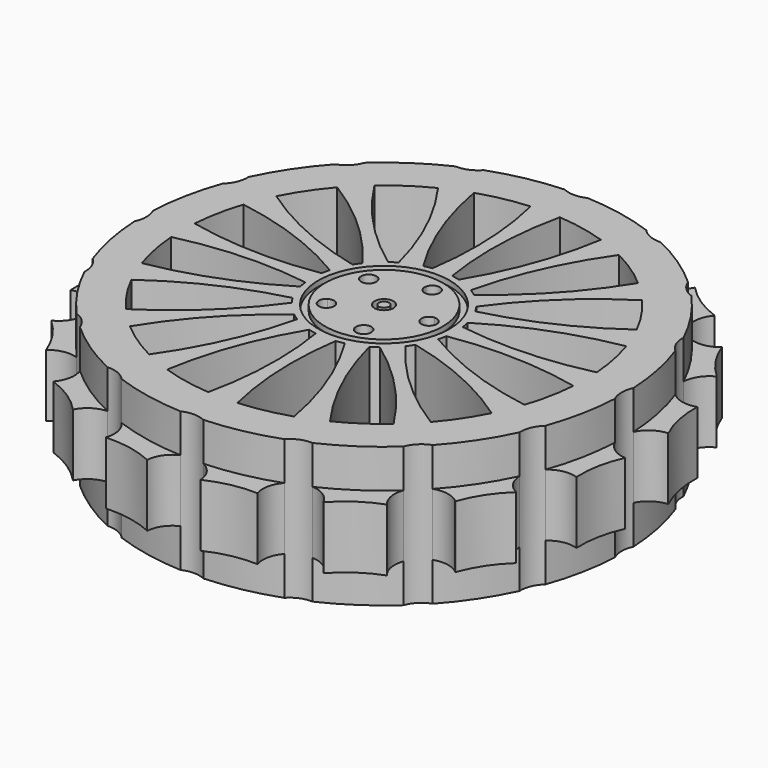
from build123d import *

# Parameters (mm, degrees)
F3_DEPTH  = 30.751
F5_DEPTH  = 20.801
F7_DEPTH  = 1.5
F6_R      = 9.7732794043
F6_R_2    = 8.7701539323
F8_DEPTH  = 0.8
F6_R_3    = 1.4109010528
F6_R_4    = 0.7822608286
F9_DEPTH  = 1.5
F10_DEPTH = 30.751


with BuildPart() as f1:
    # F0 (on Front) → F1 (revolve)
    with BuildSketch(Plane.XZ):
        Polygon((15.6630596573, 13.3769841367), (-20.1369403427, 13.3769841367), (-20.1369403427, 7.6269841367), (-18.1369403427, 7.6269841367), (-18.1369403427, -17.3730158633), (-14.1369403427, -17.3730158633), (-14.1369403427, -7.4230158633), (15.6630596573, -7.4230158633), (15.6630596573, -1.6730158633), (19.1630596573, -1.6730158633), (19.1630596573, 7.6269841367), (15.6630596573, 7.6269841367), align=None)
    revolve(axis=Axis((-20.1369403427, 0, 10.5019841367), (0, 0, -1)))

    # F2 (on face) → F3 (cut, through all)
    with BuildSketch(Plane.XY.offset(13.3769841367)):
        with BuildLine():
            ThreePointArc((18.9510825218, -3.9897850102), (19.0031496784, -3.8784203653), (19.0561068276, -3.7674761754))
            ThreePointArc((19.0561068276, -3.7674761754), (19.1915759594, -1.8859026221), (19.2367669151, 0))
            ThreePointArc((19.2367669151, 0), (19.1859387892, 2), (19.0335856412, 3.9948363383))
            ThreePointArc((19.0335856412, 3.9948363383), (19.0203353599, 3.9941403808), (19.0070874601, 3.9934004743))
            ThreePointArc((19.0070874601, 3.9934004743), (17.0018080089, 3.3173722564), (15.6220600073, 1.7128613401))
            ThreePointArc((15.6220600073, 1.7128613401), (15.652808277, 0.8566759804), (15.6630596573, 0))
            ThreePointArc((15.6630596573, 0), (15.652808277, -0.8566759804), (15.6220600073, -1.7128613401))
            ThreePointArc((15.6220600073, -1.7128613401), (16.9785910085, -3.3016119661), (18.9510825218, -3.9897850102))
        make_face()
        with BuildLine():
            ThreePointArc((19.2367669151, 0), (19.1915759594, -1.8859026221), (19.0561068276, -3.7674761754))
            ThreePointArc((19.0561068276, -3.7674761754), (19.0450111469, -3.8811725923), (19.0335856412, -3.9948363383))
            ThreePointArc((19.0335856412, -3.9948363383), (21.9924224546, -2.8993727853), (23.2367669151, 0))
            ThreePointArc((23.2367669151, 0), (21.9924224546, 2.8993727853), (19.0335856412, 3.9948363383))
            ThreePointArc((19.0335856412, 3.9948363383), (19.1859387892, 2), (19.2367669151, 0))
        make_face()
        with BuildLine():
            ThreePointArc((17.5806645732, -11.2991638023), (18.4802121707, -7.6814292279), (19.0335856412, -3.9948363383))
            ThreePointArc((19.0335856412, -3.9948363383), (18.9923210333, -3.9925237896), (18.9510825218, -3.9897850102))
            ThreePointArc((18.9510825218, -3.9897850102), (17.80492248, -7.5543523288), (17.5556339646, -11.2903499529))
            ThreePointArc((17.5556339646, -11.2903499529), (17.5681565781, -11.2947361201), (17.5806645732, -11.2991638023))
        make_face()
        with BuildLine():
            ThreePointArc((19.0070874601, 3.9934004743), (19.0203353599, 3.9941403808), (19.0335856412, 3.9948363383))
            ThreePointArc((19.0335856412, 3.9948363383), (18.4802121707, 7.6814292279), (17.5806645732, 11.2991638023))
            ThreePointArc((17.5806645732, 11.2991638023), (17.5416560725, 11.285509037), (17.5025085702, 11.2722580441))
            ThreePointArc((17.5025085702, 11.2722580441), (17.8076956231, 7.5404107973), (19.0070874601, 3.9934004743))
        make_face()
        with BuildLine():
            ThreePointArc((20.2396219119, -15.0676654384), (19.5079678731, -12.7616050147), (17.5806645732, -11.2991638023))
            ThreePointArc((17.5806645732, -11.2991638023), (16.283185196, -14.9620613209), (14.6309630405, -18.4792239437))
            ThreePointArc((14.6309630405, -18.4792239437), (14.5772022331, -18.580019603), (14.5231492098, -18.6806588598))
            ThreePointArc((14.5231492098, -18.6806588598), (18.3766887325, -18.4489293151), (20.2396219119, -15.0676654384))
        make_face()
        with BuildLine():
            ThreePointArc((14.6309630405, -18.4792239437), (16.283185196, -14.9620613209), (17.5806645732, -11.2991638023))
            ThreePointArc((17.5806645732, -11.2991638023), (17.5681565781, -11.2947361201), (17.5556339646, -11.2903499529))
            ThreePointArc((17.5556339646, -11.2903499529), (15.444292524, -11.1475313635), (13.5555518405, -12.1018994577))
            ThreePointArc((13.5555518405, -12.1018994577), (12.9379469212, -13.7000668787), (12.2445845269, -15.2668545261))
            ThreePointArc((12.2445845269, -15.2668545261), (12.8898672114, -17.2537906513), (14.448859326, -18.6444194642))
            ThreePointArc((14.448859326, -18.6444194642), (14.5395805109, -18.5614571863), (14.6309630405, -18.4792239437))
        make_face()
        with BuildLine():
            ThreePointArc((15.6220600073, 1.7128613401), (15.2367669151, 0), (15.6220600073, -1.7128613401))
            ThreePointArc((15.6220600073, -1.7128613401), (15.652808277, -0.8566759804), (15.6630596573, 0))
            ThreePointArc((15.6630596573, 0), (15.652808277, 0.8566759804), (15.6220600073, 1.7128613401))
        make_face()
        with BuildLine():
            ThreePointArc((17.5144644688, 11.5178356883), (17.5477231316, 11.4085477626), (17.5806645732, 11.2991638023))
            ThreePointArc((17.5806645732, 11.2991638023), (19.5079678731, 12.7616050147), (20.2396219119, 15.0676654384))
            ThreePointArc((20.2396219119, 15.0676654384), (18.3766887325, 18.4489293151), (14.5231492098, 18.6806588598))
            ThreePointArc((14.5231492098, 18.6806588598), (16.1957524179, 15.1731427195), (17.5144644688, 11.5178356883))
        make_face()
        with BuildLine():
            ThreePointArc((12.2445845269, -15.2668545261), (12.9379469212, -13.7000668787), (13.5555518405, -12.1018994577))
            ThreePointArc((13.5555518405, -12.1018994577), (12.5441037818, -13.5369317089), (12.2445845269, -15.2668545261))
        make_face()
        with BuildLine():
            ThreePointArc((17.5025085702, 11.2722580441), (17.507994946, 11.3950707983), (17.5144644688, 11.5178356883))
            ThreePointArc((17.5144644688, 11.5178356883), (16.1957524179, 15.1731427195), (14.5231492098, 18.6806588598))
            ThreePointArc((14.5231492098, 18.6806588598), (14.5111738775, 18.6749452158), (14.499217564, 18.6691918795))
            ThreePointArc((14.499217564, 18.6691918795), (12.9052857209, 17.2772360224), (12.2445845269, 15.2668545261))
            ThreePointArc((12.2445845269, 15.2668545261), (12.9379469212, 13.7000668787), (13.5555518405, 12.1018994577))
            ThreePointArc((13.5555518405, 12.1018994577), (15.4168116104, 11.1532072117), (17.5025085702, 11.2722580441))
        make_face()
        with BuildLine():
            ThreePointArc((10.3855800677, -24.8729686813), (12.6011007659, -21.8748597161), (14.5231492098, -18.6806588598))
            ThreePointArc((14.5231492098, -18.6806588598), (14.4859106572, -18.6627310616), (14.448859326, -18.6444194642))
            ThreePointArc((14.448859326, -18.6444194642), (12.0258446661, -21.4990337933), (10.365827715, -24.8552469469))
            ThreePointArc((10.365827715, -24.8552469469), (10.3757185877, -24.8640914338), (10.3855800677, -24.8729686813))
        make_face()
        with BuildLine():
            ThreePointArc((12.2445845269, 15.2668545261), (12.5441037818, 13.5369317089), (13.5555518405, 12.1018994577))
            ThreePointArc((13.5555518405, 12.1018994577), (12.9379469212, 13.7000668787), (12.2445845269, 15.2668545261))
        make_face()
        with BuildLine():
            ThreePointArc((14.499217564, 18.6691918795), (14.5111738775, 18.6749452158), (14.5231492098, 18.6806588598))
            ThreePointArc((14.5231492098, 18.6806588598), (12.6011007659, 21.8748597161), (10.3855800677, 24.8729686813))
            ThreePointArc((10.3855800677, 24.8729686813), (10.3547663648, 24.8454254161), (10.3236697241, 24.8182019945))
            ThreePointArc((10.3236697241, 24.8182019945), (12.0337419093, 21.4872147336), (14.499217564, 18.6691918795))
        make_face()
        with BuildLine():
            ThreePointArc((11.7044750597, -27.8414154024), (11.3599107405, -26.2172879493), (10.3855800677, -24.8729686813))
            ThreePointArc((10.3855800677, -24.8729686813), (7.7851352324, -27.7605208669), (4.9127211352, -30.3776773811))
            ThreePointArc((4.9127211352, -30.3776773811), (4.8244797967, -30.4502270574), (4.7360283386, -30.5225204104))
            ThreePointArc((4.7360283386, -30.5225204104), (9.1408268821, -31.5746302961), (11.7044750597, -27.8414154024))
        make_face()
        with BuildLine():
            ThreePointArc((4.9127211352, -30.3776773811), (7.7851352324, -27.7605208669), (10.3855800677, -24.8729686813))
            ThreePointArc((10.3855800677, -24.8729686813), (10.3757185877, -24.8640914338), (10.365827715, -24.8552469469))
            ThreePointArc((10.365827715, -24.8552469469), (8.4698568798, -23.915324386), (6.3596671621, -24.0742557671))
            ThreePointArc((6.3596671621, -24.0742557671), (5.1774824238, -25.3144227665), (3.9373154244, -26.4966075048))
            ThreePointArc((3.9373154244, -26.4966075048), (3.773111353, -28.5792361158), (4.6812616518, -30.4606100668))
            ThreePointArc((4.6812616518, -30.4606100668), (4.7968253868, -30.4186804108), (4.9127211352, -30.3776773811))
        make_face()
        with BuildLine():
            ThreePointArc((3.9373154244, -26.4966075048), (5.1774824238, -25.3144227665), (6.3596671621, -24.0742557671))
            ThreePointArc((6.3596671621, -24.0742557671), (4.876047935, -25.0129882777), (3.9373154244, -26.4966075048))
        make_face()
        with BuildLine():
            ThreePointArc((10.2407370384, 25.0496614779), (10.3132867147, 24.9614201394), (10.3855800677, 24.8729686813))
            ThreePointArc((10.3855800677, 24.8729686813), (11.3599107405, 26.2172879493), (11.7044750597, 27.8414154024))
            ThreePointArc((11.7044750597, 27.8414154024), (9.1408268821, 31.5746302961), (4.7360283386, 30.5225204104))
            ThreePointArc((4.7360283386, 30.5225204104), (7.6235805242, 27.9220755751), (10.2407370384, 25.0496614779))
        make_face()
        with BuildLine():
            ThreePointArc((3.9373154244, 26.4966075048), (5.1774824238, 25.3144227665), (6.3596671621, 24.0742557671))
            ThreePointArc((6.3596671621, 24.0742557671), (8.4422957731, 23.9100516957), (10.3236697241, 24.8182019945))
            ThreePointArc((10.3236697241, 24.8182019945), (10.2817400681, 24.9337657295), (10.2407370384, 25.0496614779))
            ThreePointArc((10.2407370384, 25.0496614779), (7.6235805242, 27.9220755751), (4.7360283386, 30.5225204104))
            ThreePointArc((4.7360283386, 30.5225204104), (4.7271510911, 30.5126589304), (4.7183066042, 30.5027680577))
            ThreePointArc((4.7183066042, 30.5027680577), (3.7783840433, 28.6067972225), (3.9373154244, 26.4966075048))
        make_face()
        with BuildLine():
            ThreePointArc((3.9373154244, 26.4966075048), (4.876047935, 25.0129882777), (6.3596671621, 24.0742557671))
            ThreePointArc((6.3596671621, 24.0742557671), (5.1774824238, 25.3144227665), (3.9373154244, 26.4966075048))
        make_face()
        with BuildLine():
            ThreePointArc((-1.4562814829, -34.6600895525), (1.7379193734, -32.7380411086), (4.7360283386, -30.5225204104))
            ThreePointArc((4.7360283386, -30.5225204104), (4.7084850734, -30.4917067075), (4.6812616518, -30.4606100668))
            ThreePointArc((4.6812616518, -30.4606100668), (1.3502743909, -32.170682252), (-1.4677484632, -34.6361579067))
            ThreePointArc((-1.4677484632, -34.6361579067), (-1.4619951269, -34.6481142202), (-1.4562814829, -34.6600895525))
        make_face()
        with BuildLine():
            ThreePointArc((-8.035040885, -33.6924921832), (-6.436873464, -33.0748872639), (-4.8700858166, -32.3815248696))
            ThreePointArc((-4.8700858166, -32.3815248696), (-6.6000086338, -32.6810441245), (-8.035040885, -33.6924921832))
        make_face()
        with BuildLine():
            ThreePointArc((-1.4677484632, -34.6361579067), (-2.8597043203, -33.0422260636), (-4.8700858166, -32.3815248696))
            ThreePointArc((-4.8700858166, -32.3815248696), (-6.436873464, -33.0748872639), (-8.035040885, -33.6924921832))
            ThreePointArc((-8.035040885, -33.6924921832), (-8.983733131, -35.5537519531), (-8.8646822986, -37.6394489129))
            ThreePointArc((-8.8646822986, -37.6394489129), (-8.7418695444, -37.6449352887), (-8.6191046544, -37.6514048115))
            ThreePointArc((-8.6191046544, -37.6514048115), (-4.9637976232, -36.3326927606), (-1.4562814829, -34.6600895525))
            ThreePointArc((-1.4562814829, -34.6600895525), (-1.4619951269, -34.6481142202), (-1.4677484632, -34.6361579067))
        make_face()
        with BuildLine():
            ThreePointArc((4.7183066042, 30.5027680577), (4.7271510911, 30.5126589304), (4.7360283386, 30.5225204104))
            ThreePointArc((4.7360283386, 30.5225204104), (1.7379193734, 32.7380411086), (-1.4562814829, 34.6600895525))
            ThreePointArc((-1.4562814829, 34.6600895525), (-1.4742092811, 34.6228509999), (-1.4925208785, 34.5857996687))
            ThreePointArc((-1.4925208785, 34.5857996687), (1.3620934506, 32.1627850088), (4.7183066042, 30.5027680577))
        make_face()
        with BuildLine():
            ThreePointArc((-1.0692749043, -36.3765622546), (-1.1672258474, -35.4967820791), (-1.4562814829, -34.6600895525))
            ThreePointArc((-1.4562814829, -34.6600895525), (-4.9637976232, -36.3326927606), (-8.6191046544, -37.6514048115))
            ThreePointArc((-8.6191046544, -37.6514048115), (-8.7283925801, -37.6846634743), (-8.8377765404, -37.7176049159))
            ThreePointArc((-8.8377765404, -37.7176049159), (-4.3888362752, -40.3182628104), (-1.0692749043, -36.3765622546))
        make_face()
        with BuildLine():
            ThreePointArc((-8.035040885, 33.6924921832), (-6.436873464, 33.0748872639), (-4.8700858166, 32.3815248696))
            ThreePointArc((-4.8700858166, 32.3815248696), (-2.8831496914, 33.0268075541), (-1.4925208785, 34.5857996687))
            ThreePointArc((-1.4925208785, 34.5857996687), (-1.5754831564, 34.6765208536), (-1.657716399, 34.7679033832))
            ThreePointArc((-1.657716399, 34.7679033832), (-5.1748790218, 36.4201255387), (-8.8377765404, 37.7176049159))
            ThreePointArc((-8.8377765404, 37.7176049159), (-8.8422042226, 37.7050969208), (-8.8465903898, 37.6925743073))
            ThreePointArc((-8.8465903898, 37.6925743073), (-8.9894089792, 35.5812328667), (-8.035040885, 33.6924921832))
        make_face()
        with BuildLine():
            ThreePointArc((-8.035040885, 33.6924921832), (-6.6000086338, 32.6810441245), (-4.8700858166, 32.3815248696))
            ThreePointArc((-4.8700858166, 32.3815248696), (-6.436873464, 33.0748872639), (-8.035040885, 33.6924921832))
        make_face()
        with BuildLine():
            ThreePointArc((-1.657716399, 34.7679033832), (-1.5569207397, 34.7141425758), (-1.4562814829, 34.6600895525))
            ThreePointArc((-1.4562814829, 34.6600895525), (-1.1672258474, 35.4967820791), (-1.0692749043, 36.3765622546))
            ThreePointArc((-1.0692749043, 36.3765622546), (-4.3888362752, 40.3182628104), (-8.8377765404, 37.7176049159))
            ThreePointArc((-8.8377765404, 37.7176049159), (-5.1748790218, 36.4201255387), (-1.657716399, 34.7679033832))
        make_face()
        with BuildLine():
            ThreePointArc((-8.8377765404, -37.7176049159), (-8.8514313057, -37.6785964152), (-8.8646822986, -37.6394489129))
            ThreePointArc((-8.8646822986, -37.6394489129), (-12.5965295454, -37.9446359658), (-16.1435398684, -39.1440278028))
            ThreePointArc((-16.1435398684, -39.1440278028), (-16.1427999619, -39.1572757026), (-16.1421040044, -39.1705259839))
            ThreePointArc((-16.1421040044, -39.1705259839), (-12.4555111148, -38.6171525134), (-8.8377765404, -37.7176049159))
        make_face()
        with BuildLine():
            ThreePointArc((-21.8498016828, -35.75900035), (-20.1369403427, -35.8), (-18.4240790026, -35.75900035))
            ThreePointArc((-18.4240790026, -35.75900035), (-20.1369403427, -35.3737072578), (-21.8498016828, -35.75900035))
        make_face()
        with BuildLine():
            ThreePointArc((-16.1435398684, -39.1440278028), (-16.8195680863, -37.1387483516), (-18.4240790026, -35.75900035))
            ThreePointArc((-18.4240790026, -35.75900035), (-20.1369403427, -35.8), (-21.8498016828, -35.75900035))
            ThreePointArc((-21.8498016828, -35.75900035), (-23.4385523088, -37.1155313512), (-24.1267253529, -39.0880228645))
            ThreePointArc((-24.1267253529, -39.0880228645), (-24.015360708, -39.1400900211), (-23.9044165181, -39.1930471703))
            ThreePointArc((-23.9044165181, -39.1930471703), (-20.022703913, -39.3735415382), (-16.1421040044, -39.1705259839))
            ThreePointArc((-16.1421040044, -39.1705259839), (-16.1427999619, -39.1572757026), (-16.1435398684, -39.1440278028))
        make_face()
        with BuildLine():
            ThreePointArc((-16.1471553325, 39.0880228645), (-12.5825880139, 37.9418628227), (-8.8465903898, 37.6925743073))
            ThreePointArc((-8.8465903898, 37.6925743073), (-8.8422042226, 37.7050969208), (-8.8377765404, 37.7176049159))
            ThreePointArc((-8.8377765404, 37.7176049159), (-12.4555111148, 38.6171525134), (-16.1421040044, 39.1705259839))
            ThreePointArc((-16.1421040044, 39.1705259839), (-16.1444165531, 39.129261376), (-16.1471553325, 39.0880228645))
        make_face()
        with BuildLine():
            ThreePointArc((-21.8498016828, 35.75900035), (-20.1369403427, 35.8), (-18.4240790026, 35.75900035))
            ThreePointArc((-18.4240790026, 35.75900035), (-16.8353283766, 37.1155313512), (-16.1471553325, 39.0880228645))
            ThreePointArc((-16.1471553325, 39.0880228645), (-16.2585199774, 39.1400900211), (-16.3694641673, 39.1930471703))
            ThreePointArc((-16.3694641673, 39.1930471703), (-20.2511767724, 39.3735415382), (-24.131776681, 39.1705259839))
            ThreePointArc((-24.131776681, 39.1705259839), (-24.1310807235, 39.1572757026), (-24.130340817, 39.1440278028))
            ThreePointArc((-24.130340817, 39.1440278028), (-23.4543125991, 37.1387483516), (-21.8498016828, 35.75900035))
        make_face()
        with BuildLine():
            ThreePointArc((-21.8498016828, 35.75900035), (-20.1369403427, 35.3737072578), (-18.4240790026, 35.75900035))
            ThreePointArc((-18.4240790026, 35.75900035), (-20.1369403427, 35.8), (-21.8498016828, 35.75900035))
        make_face()
        with BuildLine():
            ThreePointArc((-16.1369403427, -39.3737072578), (-16.1382314665, -39.2720838187), (-16.1421040044, -39.1705259839))
            ThreePointArc((-16.1421040044, -39.1705259839), (-20.022703913, -39.3735415382), (-23.9044165181, -39.1930471703))
            ThreePointArc((-23.9044165181, -39.1930471703), (-24.018112935, -39.1819514896), (-24.131776681, -39.1705259839))
            ThreePointArc((-24.131776681, -39.1705259839), (-20.2385637818, -43.372416134), (-16.1369403427, -39.3737072578))
        make_face()
        with BuildLine():
            ThreePointArc((-24.131776681, -39.1705259839), (-24.1294641323, -39.129261376), (-24.1267253529, -39.0880228645))
            ThreePointArc((-24.1267253529, -39.0880228645), (-27.6912926715, -37.9418628227), (-31.4272902956, -37.6925743073))
            ThreePointArc((-31.4272902956, -37.6925743073), (-31.4316764628, -37.7050969208), (-31.436104145, -37.7176049159))
            ThreePointArc((-31.436104145, -37.7176049159), (-27.8183695706, -38.6171525134), (-24.131776681, -39.1705259839))
        make_face()
        with BuildLine():
            ThreePointArc((-35.4037948688, -32.3815248696), (-33.8370072214, -33.0748872639), (-32.2388398004, -33.6924921832))
            ThreePointArc((-32.2388398004, -33.6924921832), (-33.6738720516, -32.6810441245), (-35.4037948688, -32.3815248696))
        make_face()
        with BuildLine():
            ThreePointArc((-31.2046057811, -36.3765622546), (-31.4721090347, -34.9383452895), (-32.2388398004, -33.6924921832))
            ThreePointArc((-32.2388398004, -33.6924921832), (-33.8370072214, -33.0748872639), (-35.4037948688, -32.3815248696))
            ThreePointArc((-35.4037948688, -32.3815248696), (-37.390730994, -33.0268075541), (-38.7813598069, -34.5857996687))
            ThreePointArc((-38.7813598069, -34.5857996687), (-38.698397529, -34.6765208536), (-38.6161642864, -34.7679033832))
            ThreePointArc((-38.6161642864, -34.7679033832), (-35.0990016636, -36.4201255387), (-31.436104145, -37.7176049159))
            ThreePointArc((-31.436104145, -37.7176049159), (-31.4316764628, -37.7050969208), (-31.4272902956, -37.6925743073))
            ThreePointArc((-31.4272902956, -37.6925743073), (-31.2606698065, -37.0439219994), (-31.2046057811, -36.3765622546))
        make_face()
        with BuildLine():
            ThreePointArc((-16.3694641673, 39.1930471703), (-16.2557677504, 39.1819514896), (-16.1421040044, 39.1705259839))
            ThreePointArc((-16.1421040044, 39.1705259839), (-16.1382314665, 39.2720838187), (-16.1369403427, 39.3737072578))
            ThreePointArc((-16.1369403427, 39.3737072578), (-20.2385637818, 43.372416134), (-24.131776681, 39.1705259839))
            ThreePointArc((-24.131776681, 39.1705259839), (-20.2511767724, 39.3735415382), (-16.3694641673, 39.1930471703))
        make_face()
        with BuildLine():
            ThreePointArc((-31.4091983868, 37.6394489129), (-27.67735114, 37.9446359658), (-24.130340817, 39.1440278028))
            ThreePointArc((-24.130340817, 39.1440278028), (-24.1310807235, 39.1572757026), (-24.131776681, 39.1705259839))
            ThreePointArc((-24.131776681, 39.1705259839), (-27.8183695706, 38.6171525134), (-31.436104145, 37.7176049159))
            ThreePointArc((-31.436104145, 37.7176049159), (-31.4224493797, 37.6785964152), (-31.4091983868, 37.6394489129))
        make_face()
        with BuildLine():
            ThreePointArc((-35.4037948688, 32.3815248696), (-33.8370072214, 33.0748872639), (-32.2388398004, 33.6924921832))
            ThreePointArc((-32.2388398004, 33.6924921832), (-31.4721090347, 34.9383452895), (-31.2046057811, 36.3765622546))
            ThreePointArc((-31.2046057811, 36.3765622546), (-31.2560851988, 37.016238119), (-31.4091983868, 37.6394489129))
            ThreePointArc((-31.4091983868, 37.6394489129), (-31.532011141, 37.6449352887), (-31.654776031, 37.6514048115))
            ThreePointArc((-31.654776031, 37.6514048115), (-35.3100830622, 36.3326927606), (-38.8175992025, 34.6600895525))
            ThreePointArc((-38.8175992025, 34.6600895525), (-38.8118855585, 34.6481142202), (-38.8061322222, 34.6361579067))
            ThreePointArc((-38.8061322222, 34.6361579067), (-37.4141763651, 33.0422260636), (-35.4037948688, 32.3815248696))
        make_face()
        with BuildLine():
            ThreePointArc((-35.4037948688, 32.3815248696), (-33.6738720516, 32.6810441245), (-32.2388398004, 33.6924921832))
            ThreePointArc((-32.2388398004, 33.6924921832), (-33.8370072214, 33.0748872639), (-35.4037948688, 32.3815248696))
        make_face()
        with BuildLine():
            ThreePointArc((-38.8175992025, -34.6600895525), (-36.7353395105, -40.0720803846), (-31.436104145, -37.7176049159))
            ThreePointArc((-31.436104145, -37.7176049159), (-35.0990016636, -36.4201255387), (-38.6161642864, -34.7679033832))
            ThreePointArc((-38.6161642864, -34.7679033832), (-38.7169599457, -34.7141425758), (-38.8175992025, -34.6600895525))
        make_face()
        with BuildLine():
            ThreePointArc((-38.8175992025, -34.6600895525), (-38.7996714043, -34.6228509999), (-38.7813598069, -34.5857996687))
            ThreePointArc((-38.7813598069, -34.5857996687), (-41.635974136, -32.1627850088), (-44.9921872896, -30.5027680577))
            ThreePointArc((-44.9921872896, -30.5027680577), (-45.0010317765, -30.5126589304), (-45.009909024, -30.5225204104))
            ThreePointArc((-45.009909024, -30.5225204104), (-42.0118000588, -32.7380411086), (-38.8175992025, -34.6600895525))
        make_face()
        with BuildLine():
            ThreePointArc((-46.6335478475, -24.0742557671), (-45.4513631092, -25.3144227665), (-44.2111961098, -26.4966075048))
            ThreePointArc((-44.2111961098, -26.4966075048), (-45.1499286204, -25.0129882777), (-46.6335478475, -24.0742557671))
        make_face()
        with BuildLine():
            ThreePointArc((-43.9783557451, -27.8414154024), (-44.0369956663, -27.1590073652), (-44.2111961098, -26.4966075048))
            ThreePointArc((-44.2111961098, -26.4966075048), (-45.4513631092, -25.3144227665), (-46.6335478475, -24.0742557671))
            ThreePointArc((-46.6335478475, -24.0742557671), (-48.7161764585, -23.9100516957), (-50.5975504095, -24.8182019945))
            ThreePointArc((-50.5975504095, -24.8182019945), (-50.5556207535, -24.9337657295), (-50.5146177238, -25.0496614779))
            ThreePointArc((-50.5146177238, -25.0496614779), (-47.8974612096, -27.9220755751), (-45.009909024, -30.5225204104))
            ThreePointArc((-45.009909024, -30.5225204104), (-45.0010317765, -30.5126589304), (-44.9921872896, -30.5027680577))
            ThreePointArc((-44.9921872896, -30.5027680577), (-44.240396822, -29.2653757562), (-43.9783557451, -27.8414154024))
        make_face()
        with BuildLine():
            ThreePointArc((-31.654776031, 37.6514048115), (-31.5454881053, 37.6846634743), (-31.436104145, 37.7176049159))
            ThreePointArc((-31.436104145, 37.7176049159), (-36.7353395105, 40.0720803846), (-38.8175992025, 34.6600895525))
            ThreePointArc((-38.8175992025, 34.6600895525), (-35.3100830622, 36.3326927606), (-31.654776031, 37.6514048115))
        make_face()
        with BuildLine():
            ThreePointArc((-44.9551423372, 30.4606100668), (-41.6241550763, 32.170682252), (-38.8061322222, 34.6361579067))
            ThreePointArc((-38.8061322222, 34.6361579067), (-38.8118855585, 34.6481142202), (-38.8175992025, 34.6600895525))
            ThreePointArc((-38.8175992025, 34.6600895525), (-42.0118000588, 32.7380411086), (-45.009909024, 30.5225204104))
            ThreePointArc((-45.009909024, 30.5225204104), (-44.9823657588, 30.4917067075), (-44.9551423372, 30.4606100668))
        make_face()
        with BuildLine():
            ThreePointArc((-46.6335478475, 24.0742557671), (-45.4513631092, 25.3144227665), (-44.2111961098, 26.4966075048))
            ThreePointArc((-44.2111961098, 26.4966075048), (-44.0369956663, 27.1590073652), (-43.9783557451, 27.8414154024))
            ThreePointArc((-43.9783557451, 27.8414154024), (-44.2304994491, 29.2391182264), (-44.9551423372, 30.4606100668))
            ThreePointArc((-44.9551423372, 30.4606100668), (-45.0707060722, 30.4186804108), (-45.1866018206, 30.3776773811))
            ThreePointArc((-45.1866018206, 30.3776773811), (-48.0590159178, 27.7605208669), (-50.6594607531, 24.8729686813))
            ThreePointArc((-50.6594607531, 24.8729686813), (-50.6495992731, 24.8640914338), (-50.6397084004, 24.8552469469))
            ThreePointArc((-50.6397084004, 24.8552469469), (-48.7437375652, 23.915324386), (-46.6335478475, 24.0742557671))
        make_face()
        with BuildLine():
            ThreePointArc((-46.6335478475, 24.0742557671), (-45.1499286204, 25.0129882777), (-44.2111961098, 26.4966075048))
            ThreePointArc((-44.2111961098, 26.4966075048), (-45.4513631092, 25.3144227665), (-46.6335478475, 24.0742557671))
        make_face()
        with BuildLine():
            ThreePointArc((-50.6594607531, -24.8729686813), (-50.8067828699, -30.6698425272), (-45.009909024, -30.5225204104))
            ThreePointArc((-45.009909024, -30.5225204104), (-47.8974612096, -27.9220755751), (-50.5146177238, -25.0496614779))
            ThreePointArc((-50.5146177238, -25.0496614779), (-50.5871674001, -24.9614201394), (-50.6594607531, -24.8729686813))
        make_face()
        with BuildLine():
            ThreePointArc((-50.6594607531, -24.8729686813), (-50.6286470502, -24.8454254161), (-50.5975504095, -24.8182019945))
            ThreePointArc((-50.5975504095, -24.8182019945), (-52.3076225947, -21.4872147336), (-54.7730982494, -18.6691918795))
            ThreePointArc((-54.7730982494, -18.6691918795), (-54.7850545629, -18.6749452158), (-54.7970298952, -18.6806588598))
            ThreePointArc((-54.7970298952, -18.6806588598), (-52.8749814513, -21.8748597161), (-50.6594607531, -24.8729686813))
        make_face()
        with BuildLine():
            ThreePointArc((-53.8294325259, -12.1018994577), (-53.2118276066, -13.7000668787), (-52.5184652123, -15.2668545261))
            ThreePointArc((-52.5184652123, -15.2668545261), (-52.5147434435, -15.1672908872), (-52.5135025973, -15.0676654384))
            ThreePointArc((-52.5135025973, -15.0676654384), (-52.8572558684, -13.4453646471), (-53.8294325259, -12.1018994577))
        make_face()
        with BuildLine():
            ThreePointArc((-54.7730982494, -18.6691918795), (-53.1791664063, -17.2772360224), (-52.5184652123, -15.2668545261))
            ThreePointArc((-52.5184652123, -15.2668545261), (-53.2118276066, -13.7000668787), (-53.8294325259, -12.1018994577))
            ThreePointArc((-53.8294325259, -12.1018994577), (-55.6906922958, -11.1532072117), (-57.7763892556, -11.2722580441))
            ThreePointArc((-57.7763892556, -11.2722580441), (-57.7818756314, -11.3950707983), (-57.7883451542, -11.5178356883))
            ThreePointArc((-57.7883451542, -11.5178356883), (-56.4696331033, -15.1731427195), (-54.7970298952, -18.6806588598))
            ThreePointArc((-54.7970298952, -18.6806588598), (-54.7850545629, -18.6749452158), (-54.7730982494, -18.6691918795))
        make_face()
        with BuildLine():
            ThreePointArc((-45.1866018206, 30.3776773811), (-45.0983604821, 30.4502270574), (-45.009909024, 30.5225204104))
            ThreePointArc((-45.009909024, 30.5225204104), (-50.8067828699, 30.6698425272), (-50.6594607531, 24.8729686813))
            ThreePointArc((-50.6594607531, 24.8729686813), (-48.0590159178, 27.7605208669), (-45.1866018206, 30.3776773811))
        make_face()
        with BuildLine():
            ThreePointArc((-54.7227400114, 18.6444194642), (-52.2997253515, 21.4990337933), (-50.6397084004, 24.8552469469))
            ThreePointArc((-50.6397084004, 24.8552469469), (-50.6495992731, 24.8640914338), (-50.6594607531, 24.8729686813))
            ThreePointArc((-50.6594607531, 24.8729686813), (-52.8749814513, 21.8748597161), (-54.7970298952, 18.6806588598))
            ThreePointArc((-54.7970298952, 18.6806588598), (-54.7597913426, 18.6627310616), (-54.7227400114, 18.6444194642))
        make_face()
        with BuildLine():
            ThreePointArc((-53.8294325259, 12.1018994577), (-53.2118276066, 13.7000668787), (-52.5184652123, 15.2668545261))
            ThreePointArc((-52.5184652123, 15.2668545261), (-53.1637478968, 17.2537906513), (-54.7227400114, 18.6444194642))
            ThreePointArc((-54.7227400114, 18.6444194642), (-54.8134611963, 18.5614571863), (-54.9048437259, 18.4792239437))
            ThreePointArc((-54.9048437259, 18.4792239437), (-56.5570658814, 14.9620613209), (-57.8545452586, 11.2991638023))
            ThreePointArc((-57.8545452586, 11.2991638023), (-57.8420372635, 11.2947361201), (-57.82951465, 11.2903499529))
            ThreePointArc((-57.82951465, 11.2903499529), (-55.7181732094, 11.1475313635), (-53.8294325259, 12.1018994577))
        make_face()
        with BuildLine():
            ThreePointArc((-52.5135025973, 15.0676654384), (-52.5147434435, 15.1672908872), (-52.5184652123, 15.2668545261))
            ThreePointArc((-52.5184652123, 15.2668545261), (-53.2118276066, 13.7000668787), (-53.8294325259, 12.1018994577))
            ThreePointArc((-53.8294325259, 12.1018994577), (-52.8572558684, 13.4453646471), (-52.5135025973, 15.0676654384))
        make_face()
        with BuildLine():
            ThreePointArc((-57.8545452586, -11.2991638023), (-60.2090207273, -16.5983991678), (-54.7970298952, -18.6806588598))
            ThreePointArc((-54.7970298952, -18.6806588598), (-56.4696331033, -15.1731427195), (-57.7883451542, -11.5178356883))
            ThreePointArc((-57.7883451542, -11.5178356883), (-57.821603817, -11.4085477626), (-57.8545452586, -11.2991638023))
        make_face()
        with BuildLine():
            ThreePointArc((-57.8545452586, -11.2991638023), (-57.8155367579, -11.285509037), (-57.7763892556, -11.2722580441))
            ThreePointArc((-57.7763892556, -11.2722580441), (-58.0815763085, -7.5404107973), (-59.2809681455, -3.9934004743))
            ThreePointArc((-59.2809681455, -3.9934004743), (-59.2942160453, -3.9941403808), (-59.3074663266, -3.9948363383))
            ThreePointArc((-59.3074663266, -3.9948363383), (-58.7540928561, -7.6814292279), (-57.8545452586, -11.2991638023))
        make_face()
        with BuildLine():
            ThreePointArc((-55.8959406927, 1.7128613401), (-55.9369403427, 0), (-55.8959406927, -1.7128613401))
            ThreePointArc((-55.8959406927, -1.7128613401), (-55.6081594435, -0.8778303847), (-55.5106476005, 0))
            ThreePointArc((-55.5106476005, 0), (-55.6081594435, 0.8778303847), (-55.8959406927, 1.7128613401))
        make_face()
        with BuildLine():
            ThreePointArc((-59.2809681455, -3.9934004743), (-57.2756886943, -3.3173722564), (-55.8959406927, -1.7128613401))
            ThreePointArc((-55.8959406927, -1.7128613401), (-55.9369403427, 0), (-55.8959406927, 1.7128613401))
            ThreePointArc((-55.8959406927, 1.7128613401), (-57.2524716939, 3.3016119661), (-59.2249632072, 3.9897850102))
            ThreePointArc((-59.2249632072, 3.9897850102), (-59.2770303638, 3.8784203653), (-59.329987513, 3.7674761754))
            ThreePointArc((-59.329987513, 3.7674761754), (-59.5104818809, -0.1142364297), (-59.3074663266, -3.9948363383))
            ThreePointArc((-59.3074663266, -3.9948363383), (-59.2942160453, -3.9941403808), (-59.2809681455, -3.9934004743))
        make_face()
        with BuildLine():
            ThreePointArc((-54.9048437259, 18.4792239437), (-54.8510829185, 18.580019603), (-54.7970298952, 18.6806588598))
            ThreePointArc((-54.7970298952, 18.6806588598), (-60.2090207273, 16.5983991678), (-57.8545452586, 11.2991638023))
            ThreePointArc((-57.8545452586, 11.2991638023), (-56.5570658814, 14.9620613209), (-54.9048437259, 18.4792239437))
        make_face()
        with BuildLine():
            ThreePointArc((-59.2249632072, 3.9897850102), (-58.0788031654, 7.5543523288), (-57.82951465, 11.2903499529))
            ThreePointArc((-57.82951465, 11.2903499529), (-57.8420372635, 11.2947361201), (-57.8545452586, 11.2991638023))
            ThreePointArc((-57.8545452586, 11.2991638023), (-58.7540928561, 7.6814292279), (-59.3074663266, 3.9948363383))
            ThreePointArc((-59.3074663266, 3.9948363383), (-59.2662017187, 3.9925237896), (-59.2249632072, 3.9897850102))
        make_face()
        with BuildLine():
            ThreePointArc((-59.3074663266, 3.9948363383), (-63.5106476005, 0), (-59.3074663266, -3.9948363383))
            ThreePointArc((-59.3074663266, -3.9948363383), (-59.5104818809, -0.1142364297), (-59.329987513, 3.7674761754))
            ThreePointArc((-59.329987513, 3.7674761754), (-59.3188918323, 3.8811725923), (-59.3074663266, 3.9948363383))
        make_face()
    extrude(amount=-F3_DEPTH, mode=Mode.SUBTRACT)

    # F4 (on face) → F5 (cut, through all)
    with BuildSketch(Plane(origin=(0, 0, -7.4230158633), x_dir=(1, 0, 0), z_dir=(0, 0, -1))):
        with BuildLine():
            ThreePointArc((-11.6660608479, 6.6032522858), (-11.3052466368, 6.1122766994), (-10.9728543085, 5.6016307735))
            ThreePointArc((-10.9728543085, 5.6016307735), (-1.7575267031, 8.7043382506), (6.6978225975, 13.5060176204))
            ThreePointArc((6.6978225975, 13.5060176204), (4.8243988213, 16.7167150229), (2.5687959513, 19.6714654605))
            ThreePointArc((2.5687959513, 19.6714654605), (-5.1757327792, 13.8204425733), (-11.6660608479, 6.6032522858))
        make_face()
        with BuildLine():
            ThreePointArc((-9.7839129056, 2.8589443946), (-9.6384522635, 2.2672644786), (-9.5267775303, 1.6682881223))
            ThreePointArc((-9.5267775303, 1.6682881223), (0.1744297767, 1.0082628574), (9.8236770781, 2.2087140565))
            ThreePointArc((9.8236770781, 2.2087140565), (9.3215398978, 5.8919399127), (8.368368612, 9.484955214))
            ThreePointArc((8.368368612, 9.484955214), (-1.0257324924, 7.043017761), (-9.7839129056, 2.8589443946))
        make_face()
        with BuildLine():
            ThreePointArc((9.8282663856, -2.1455534824), (0.2147596427, -0.8066426603), (-9.4779195402, -1.3206118642))
            ThreePointArc((-9.4779195402, -1.3206118642), (-9.5699575313, -1.9229182062), (-9.6960018589, -2.5190362725))
            ThreePointArc((-9.6960018589, -2.5190362725), (-0.9858357211, -6.841311416), (8.38829915, -9.4248462004))
            ThreePointArc((8.38829915, -9.4248462004), (9.3338943995, -5.8298296385), (9.8282663856, -2.1455534824))
        make_face()
        with BuildLine():
            ThreePointArc((6.7262330701, -13.4494211106), (-1.6431100563, -8.5334990488), (-10.7946654676, -5.2991169381))
            ThreePointArc((-10.7946654676, -5.2991169381), (-11.1101901421, -5.8203540254), (-11.4547644243, -6.3228602299))
            ThreePointArc((-11.4547644243, -6.3228602299), (-5.0616832924, -13.649358043), (2.6102120911, -19.6235590597))
            ThreePointArc((2.6102120911, -19.6235590597), (4.8595814655, -16.6640604749), (6.7262330701, -13.4494211106))
        make_face()
        with BuildLine():
            ThreePointArc((-0.4654748822, -22.705736294), (-6.3164977694, -14.9612075635), (-13.5336880569, -8.4708794948))
            ThreePointArc((-13.5336880569, -8.4708794948), (-14.0246636433, -8.8316937059), (-14.5353095692, -9.1640860342))
            ThreePointArc((-14.5353095692, -9.1640860342), (-11.4326020921, -18.3794136396), (-6.6309227223, -26.8347629402))
            ThreePointArc((-6.6309227223, -26.8347629402), (-3.4202253198, -24.961339164), (-0.4654748822, -22.705736294))
        make_face()
        with BuildLine():
            ThreePointArc((-10.6519851287, -28.5053089547), (-13.0939225817, -19.1112078503), (-17.2779959481, -10.3530274371))
            ThreePointArc((-17.2779959481, -10.3530274371), (-17.8696758641, -10.4984880792), (-18.4686522204, -10.6101628124))
            ThreePointArc((-18.4686522204, -10.6101628124), (-19.1286774853, -20.3113701194), (-17.9282262862, -29.9606174208))
            ThreePointArc((-17.9282262862, -29.9606174208), (-14.24500043, -29.4584802405), (-10.6519851287, -28.5053089547))
        make_face()
        with BuildLine():
            ThreePointArc((-22.2824938251, -29.9652067283), (-20.943583003, -20.3516999854), (-21.4575522069, -10.6590208025))
            ThreePointArc((-21.4575522069, -10.6590208025), (-22.0598585489, -10.5669828114), (-22.6559766152, -10.4409384838))
            ThreePointArc((-22.6559766152, -10.4409384838), (-26.9782517587, -19.1511046216), (-29.5617865431, -28.5252394927))
            ThreePointArc((-29.5617865431, -28.5252394927), (-25.9667699812, -29.4708347422), (-22.2824938251, -29.9652067283))
        make_face()
        with BuildLine():
            ThreePointArc((-42.8426766367, -19.6714654605), (-35.0981479062, -13.8204425733), (-28.6078198375, -6.6032522858))
            ThreePointArc((-28.6078198375, -6.6032522858), (-28.9686340486, -6.1122766994), (-29.3010263769, -5.6016307735))
            ThreePointArc((-29.3010263769, -5.6016307735), (-38.5163539823, -8.7043382506), (-46.9717032829, -13.5060176204))
            ThreePointArc((-46.9717032829, -13.5060176204), (-45.0982795067, -16.7167150229), (-42.8426766367, -19.6714654605))
        make_face()
        with BuildLine():
            ThreePointArc((-48.6422492974, -9.484955214), (-39.248148193, -7.043017761), (-30.4899677798, -2.8589443946))
            ThreePointArc((-30.4899677798, -2.8589443946), (-30.6354284219, -2.2672644786), (-30.7471031551, -1.6682881223))
            ThreePointArc((-30.7471031551, -1.6682881223), (-40.4483104621, -1.0082628574), (-50.0975577635, -2.2087140565))
            ThreePointArc((-50.0975577635, -2.2087140565), (-49.5954205832, -5.8919399127), (-48.6422492974, -9.484955214))
        make_face()
        with BuildLine():
            ThreePointArc((-30.7959611452, 1.3206118642), (-30.7039231541, 1.9229182062), (-30.5778788265, 2.5190362725))
            ThreePointArc((-30.5778788265, 2.5190362725), (-39.2880449643, 6.841311416), (-48.6621798354, 9.4248462004))
            ThreePointArc((-48.6621798354, 9.4248462004), (-49.6077750849, 5.8298296385), (-50.102147071, 2.1455534824))
            ThreePointArc((-50.102147071, 2.1455534824), (-40.4886403281, 0.8066426603), (-30.7959611452, 1.3206118642))
        make_face()
        with BuildLine():
            ThreePointArc((-33.5863614533, -26.8631734128), (-28.6704393915, -18.4938302864), (-25.4360572808, -9.3422748751))
            ThreePointArc((-25.4360572808, -9.3422748751), (-25.9572943681, -9.0267502006), (-26.4598005726, -8.6821759184))
            ThreePointArc((-26.4598005726, -8.6821759184), (-33.7862983857, -15.0752570503), (-39.7604994024, -22.7471524338))
            ThreePointArc((-39.7604994024, -22.7471524338), (-36.8010008176, -24.9965218082), (-33.5863614533, -26.8631734128))
        make_face()
        with BuildLine():
            ThreePointArc((-29.4792152178, 5.2991169381), (-29.1636905433, 5.8203540254), (-28.8191162611, 6.3228602299))
            ThreePointArc((-28.8191162611, 6.3228602299), (-35.212197393, 13.649358043), (-42.8840927765, 19.6235590597))
            ThreePointArc((-42.8840927765, 19.6235590597), (-45.1334621509, 16.6640604749), (-47.0001137555, 13.4494211106))
            ThreePointArc((-47.0001137555, 13.4494211106), (-38.6307706291, 8.5334990488), (-29.4792152178, 5.2991169381))
        make_face()
        with BuildLine():
            ThreePointArc((-26.7401926285, 8.4708794948), (-26.2492170421, 8.8316937059), (-25.7385711162, 9.1640860342))
            ThreePointArc((-25.7385711162, 9.1640860342), (-28.8412785933, 18.3794136396), (-33.6429579631, 26.8347629402))
            ThreePointArc((-33.6429579631, 26.8347629402), (-36.8536553656, 24.961339164), (-39.8084058032, 22.705736294))
            ThreePointArc((-39.8084058032, 22.705736294), (-33.957382916, 14.9612075635), (-26.7401926285, 8.4708794948))
        make_face()
        with BuildLine():
            ThreePointArc((-22.9958847373, 10.3530274371), (-22.4042048213, 10.4984880792), (-21.805228465, 10.6101628124))
            ThreePointArc((-21.805228465, 10.6101628124), (-21.1452032001, 20.3113701194), (-22.3456543992, 29.9606174208))
            ThreePointArc((-22.3456543992, 29.9606174208), (-26.0288802554, 29.4584802405), (-29.6218955567, 28.5053089547))
            ThreePointArc((-29.6218955567, 28.5053089547), (-27.1799581037, 19.1112078503), (-22.9958847373, 10.3530274371))
        make_face()
        with BuildLine():
            ThreePointArc((-18.8163284785, 10.6590208025), (-18.2140221365, 10.5669828114), (-17.6179040702, 10.4409384838))
            ThreePointArc((-17.6179040702, 10.4409384838), (-13.2956289267, 19.1511046216), (-10.7120941424, 28.5252394927))
            ThreePointArc((-10.7120941424, 28.5252394927), (-14.3071107042, 29.4708347422), (-17.9913868603, 29.9652067283))
            ThreePointArc((-17.9913868603, 29.9652067283), (-19.3302976824, 20.3516999854), (-18.8163284785, 10.6590208025))
        make_face()
        with BuildLine():
            ThreePointArc((-14.8378234046, 9.3422748751), (-14.3165863173, 9.0267502006), (-13.8140801128, 8.6821759184))
            ThreePointArc((-13.8140801128, 8.6821759184), (-6.4875822997, 15.0752570503), (-0.513381283, 22.7471524338))
            ThreePointArc((-0.513381283, 22.7471524338), (-3.4728798678, 24.9965218082), (-6.6875192321, 26.8631734128))
            ThreePointArc((-6.6875192321, 26.8631734128), (-11.6034412939, 18.4938302864), (-14.8378234046, 9.3422748751))
        make_face()
    extrude(amount=-F5_DEPTH, mode=Mode.SUBTRACT)

    # F6 (on face) → F7 (cut)
    with BuildSketch(Plane.XY.offset(13.3769841367)):
        with BuildLine():
            ThreePointArc((-26.1477993657, 2.9672449234), (-25.5600684796, 3.9401332263), (-24.8164155515, 4.7997375346))
            ThreePointArc((-24.8164155515, 4.7997375346), (-26.4796255541, 4.6082305478), (-26.1477993657, 2.9672449234))
        make_face()
        with BuildLine():
            ThreePointArc((-19.1723803117, 6.6335957502), (-18.0654897197, 6.3752694803), (-17.0181560482, 5.9336458569))
            ThreePointArc((-17.0181560482, 5.9336458569), (-16.95140368, 6.1499884549), (-16.9288546665, 6.3752694803))
            ThreePointArc((-16.9288546665, 6.3752694803), (-17.9354731875, 7.5044439335), (-19.1723803117, 6.6335957502))
        make_face()
        with BuildLine():
            ThreePointArc((-19.1723803117, 6.6335957502), (-18.4167292676, 5.2942653063), (-17.0181560482, 5.9336458569))
            ThreePointArc((-17.0181560482, 5.9336458569), (-18.0654897197, 6.3752694803), (-19.1723803117, 6.6335957502))
        make_face()
        with BuildLine():
            ThreePointArc((-13.5299504364, -1.1325427178), (-13.4577200425, -0.5683175266), (-13.4335853148, 0))
            ThreePointArc((-13.4335853148, 0), (-13.4577200425, 0.5683175266), (-13.5299504364, 1.1325427178))
            ThreePointArc((-13.5299504364, 1.1325427178), (-14.5702203681, 0), (-13.5299504364, -1.1325427178))
        make_face()
        with BuildLine():
            ThreePointArc((-13.5299504364, 1.1325427178), (-13.4577200425, 0.5683175266), (-13.4335853148, 0))
            ThreePointArc((-13.4335853148, 0), (-13.4577200425, -0.5683175266), (-13.5299504364, -1.1325427178))
            ThreePointArc((-13.5299504364, -1.1325427178), (-12.6646876398, -0.837099522), (-12.2969502615, 0))
            ThreePointArc((-12.2969502615, 0), (-12.6646876398, 0.837099522), (-13.5299504364, 1.1325427178))
        make_face()
        with BuildLine():
            ThreePointArc((-19.1723803117, -6.6335957502), (-18.0654897197, -6.3752694803), (-17.0181560482, -5.9336458569))
            ThreePointArc((-17.0181560482, -5.9336458569), (-18.4167292676, -5.2942653063), (-19.1723803117, -6.6335957502))
        make_face()
        with BuildLine():
            ThreePointArc((-16.9288546665, -6.3752694803), (-16.95140368, -6.1499884549), (-17.0181560482, -5.9336458569))
            ThreePointArc((-17.0181560482, -5.9336458569), (-18.0654897197, -6.3752694803), (-19.1723803117, -6.6335957502))
            ThreePointArc((-19.1723803117, -6.6335957502), (-17.9354731875, -7.5044439335), (-16.9288546665, -6.3752694803))
        make_face()
        with BuildLine():
            ThreePointArc((-26.1477993657, -2.9672449234), (-25.5600684796, -3.9401332263), (-24.8164155515, -4.7997375346))
            ThreePointArc((-24.8164155515, -4.7997375346), (-24.5263370759, -4.4127203922), (-24.4234334263, -3.9401332263))
            ThreePointArc((-24.4234334263, -3.9401332263), (-25.0015419729, -2.9501901038), (-26.1477993657, -2.9672449234))
        make_face()
        with BuildLine():
            ThreePointArc((-26.1477993657, -2.9672449234), (-26.4796255541, -4.6082305478), (-24.8164155515, -4.7997375346))
            ThreePointArc((-24.8164155515, -4.7997375346), (-25.5600684796, -3.9401332263), (-26.1477993657, -2.9672449234))
        make_face()
        with BuildLine():
            ThreePointArc((-24.4234334263, 3.9401332263), (-24.5263370759, 4.4127203922), (-24.8164155515, 4.7997375346))
            ThreePointArc((-24.8164155515, 4.7997375346), (-25.5600684796, 3.9401332263), (-26.1477993657, 2.9672449234))
            ThreePointArc((-26.1477993657, 2.9672449234), (-25.0015419729, 2.9501901038), (-24.4234334263, 3.9401332263))
        make_face()
    extrude(amount=-F7_DEPTH, mode=Mode.SUBTRACT)

    # F6 (on face) → F8 (cut)
    with BuildSketch(Plane.XY.offset(13.3769841367)):
        with Locations((-20.1369403427, 0)):
            Circle(F6_R)
        with Locations((-20.1369403427, 0)):
            Circle(F6_R_2, mode=Mode.SUBTRACT)
    extrude(amount=-F8_DEPTH, mode=Mode.SUBTRACT)

    # F6 (on face) → F9 (cut)
    with BuildSketch(Plane.XY.offset(13.3769841367)):
        with Locations((-20.1369403427, 0)):
            Circle(F6_R_3)
        with Locations((-20.1369403427, 0)):
            Circle(F6_R_4, mode=Mode.SUBTRACT)
    extrude(amount=-F9_DEPTH, mode=Mode.SUBTRACT)

    # F2 (on face) → F10 (cut, through all)
    with BuildSketch(Plane.XY.offset(13.3769841367)):
        with BuildLine():
            ThreePointArc((14.5231492098, -18.6806588598), (14.5772022331, -18.580019603), (14.6309630405, -18.4792239437))
            ThreePointArc((14.6309630405, -18.4792239437), (14.5395805109, -18.5614571863), (14.448859326, -18.6444194642))
            ThreePointArc((14.448859326, -18.6444194642), (14.4859106572, -18.6627310616), (14.5231492098, -18.6806588598))
        make_face()
        with BuildLine():
            ThreePointArc((20.2396219119, -15.0676654384), (19.5079678731, -12.7616050147), (17.5806645732, -11.2991638023))
            ThreePointArc((17.5806645732, -11.2991638023), (16.283185196, -14.9620613209), (14.6309630405, -18.4792239437))
            ThreePointArc((14.6309630405, -18.4792239437), (14.5772022331, -18.580019603), (14.5231492098, -18.6806588598))
            ThreePointArc((14.5231492098, -18.6806588598), (18.3766887325, -18.4489293151), (20.2396219119, -15.0676654384))
        make_face()
        with BuildLine():
            ThreePointArc((19.0335856412, -3.9948363383), (19.0450111469, -3.8811725923), (19.0561068276, -3.7674761754))
            ThreePointArc((19.0561068276, -3.7674761754), (19.0031496784, -3.8784203653), (18.9510825218, -3.9897850102))
            ThreePointArc((18.9510825218, -3.9897850102), (18.9923210333, -3.9925237896), (19.0335856412, -3.9948363383))
        make_face()
        with BuildLine():
            ThreePointArc((17.5806645732, -11.2991638023), (18.4802121707, -7.6814292279), (19.0335856412, -3.9948363383))
            ThreePointArc((19.0335856412, -3.9948363383), (18.9923210333, -3.9925237896), (18.9510825218, -3.9897850102))
            ThreePointArc((18.9510825218, -3.9897850102), (17.80492248, -7.5543523288), (17.5556339646, -11.2903499529))
            ThreePointArc((17.5556339646, -11.2903499529), (17.5681565781, -11.2947361201), (17.5806645732, -11.2991638023))
        make_face()
        with BuildLine():
            ThreePointArc((18.9510825218, -3.9897850102), (19.0031496784, -3.8784203653), (19.0561068276, -3.7674761754))
            ThreePointArc((19.0561068276, -3.7674761754), (19.1915759594, -1.8859026221), (19.2367669151, 0))
            ThreePointArc((19.2367669151, 0), (19.1859387892, 2), (19.0335856412, 3.9948363383))
            ThreePointArc((19.0335856412, 3.9948363383), (19.0203353599, 3.9941403808), (19.0070874601, 3.9934004743))
            ThreePointArc((19.0070874601, 3.9934004743), (17.0018080089, 3.3173722564), (15.6220600073, 1.7128613401))
            ThreePointArc((15.6220600073, 1.7128613401), (15.652808277, 0.8566759804), (15.6630596573, 0))
            ThreePointArc((15.6630596573, 0), (15.652808277, -0.8566759804), (15.6220600073, -1.7128613401))
            ThreePointArc((15.6220600073, -1.7128613401), (16.9785910085, -3.3016119661), (18.9510825218, -3.9897850102))
        make_face()
        with BuildLine():
            ThreePointArc((19.2367669151, 0), (19.1915759594, -1.8859026221), (19.0561068276, -3.7674761754))
            ThreePointArc((19.0561068276, -3.7674761754), (19.0450111469, -3.8811725923), (19.0335856412, -3.9948363383))
            ThreePointArc((19.0335856412, -3.9948363383), (21.9924224546, -2.8993727853), (23.2367669151, 0))
            ThreePointArc((23.2367669151, 0), (21.9924224546, 2.8993727853), (19.0335856412, 3.9948363383))
            ThreePointArc((19.0335856412, 3.9948363383), (19.1859387892, 2), (19.2367669151, 0))
        make_face()
        with BuildLine():
            ThreePointArc((17.5144644688, 11.5178356883), (17.5477231316, 11.4085477626), (17.5806645732, 11.2991638023))
            ThreePointArc((17.5806645732, 11.2991638023), (19.5079678731, 12.7616050147), (20.2396219119, 15.0676654384))
            ThreePointArc((20.2396219119, 15.0676654384), (18.3766887325, 18.4489293151), (14.5231492098, 18.6806588598))
            ThreePointArc((14.5231492098, 18.6806588598), (16.1957524179, 15.1731427195), (17.5144644688, 11.5178356883))
        make_face()
        with BuildLine():
            ThreePointArc((17.5025085702, 11.2722580441), (17.5416560725, 11.285509037), (17.5806645732, 11.2991638023))
            ThreePointArc((17.5806645732, 11.2991638023), (17.5477231316, 11.4085477626), (17.5144644688, 11.5178356883))
            ThreePointArc((17.5144644688, 11.5178356883), (17.507994946, 11.3950707983), (17.5025085702, 11.2722580441))
        make_face()
        with BuildLine():
            ThreePointArc((10.3236697241, 24.8182019945), (10.3547663648, 24.8454254161), (10.3855800677, 24.8729686813))
            ThreePointArc((10.3855800677, 24.8729686813), (10.3132867147, 24.9614201394), (10.2407370384, 25.0496614779))
            ThreePointArc((10.2407370384, 25.0496614779), (10.2817400681, 24.9337657295), (10.3236697241, 24.8182019945))
        make_face()
        with BuildLine():
            ThreePointArc((14.499217564, 18.6691918795), (14.5111738775, 18.6749452158), (14.5231492098, 18.6806588598))
            ThreePointArc((14.5231492098, 18.6806588598), (12.6011007659, 21.8748597161), (10.3855800677, 24.8729686813))
            ThreePointArc((10.3855800677, 24.8729686813), (10.3547663648, 24.8454254161), (10.3236697241, 24.8182019945))
            ThreePointArc((10.3236697241, 24.8182019945), (12.0337419093, 21.4872147336), (14.499217564, 18.6691918795))
        make_face()
        with BuildLine():
            ThreePointArc((19.0070874601, 3.9934004743), (19.0203353599, 3.9941403808), (19.0335856412, 3.9948363383))
            ThreePointArc((19.0335856412, 3.9948363383), (18.4802121707, 7.6814292279), (17.5806645732, 11.2991638023))
            ThreePointArc((17.5806645732, 11.2991638023), (17.5416560725, 11.285509037), (17.5025085702, 11.2722580441))
            ThreePointArc((17.5025085702, 11.2722580441), (17.8076956231, 7.5404107973), (19.0070874601, 3.9934004743))
        make_face()
        with BuildLine():
            ThreePointArc((10.2407370384, 25.0496614779), (10.3132867147, 24.9614201394), (10.3855800677, 24.8729686813))
            ThreePointArc((10.3855800677, 24.8729686813), (11.3599107405, 26.2172879493), (11.7044750597, 27.8414154024))
            ThreePointArc((11.7044750597, 27.8414154024), (9.1408268821, 31.5746302961), (4.7360283386, 30.5225204104))
            ThreePointArc((4.7360283386, 30.5225204104), (7.6235805242, 27.9220755751), (10.2407370384, 25.0496614779))
        make_face()
        with BuildLine():
            ThreePointArc((-1.4925208785, 34.5857996687), (-1.4742092811, 34.6228509999), (-1.4562814829, 34.6600895525))
            ThreePointArc((-1.4562814829, 34.6600895525), (-1.5569207397, 34.7141425758), (-1.657716399, 34.7679033832))
            ThreePointArc((-1.657716399, 34.7679033832), (-1.5754831564, 34.6765208536), (-1.4925208785, 34.5857996687))
        make_face()
        with BuildLine():
            ThreePointArc((4.7183066042, 30.5027680577), (4.7271510911, 30.5126589304), (4.7360283386, 30.5225204104))
            ThreePointArc((4.7360283386, 30.5225204104), (1.7379193734, 32.7380411086), (-1.4562814829, 34.6600895525))
            ThreePointArc((-1.4562814829, 34.6600895525), (-1.4742092811, 34.6228509999), (-1.4925208785, 34.5857996687))
            ThreePointArc((-1.4925208785, 34.5857996687), (1.3620934506, 32.1627850088), (4.7183066042, 30.5027680577))
        make_face()
        with BuildLine():
            ThreePointArc((-1.657716399, 34.7679033832), (-1.5569207397, 34.7141425758), (-1.4562814829, 34.6600895525))
            ThreePointArc((-1.4562814829, 34.6600895525), (-1.1672258474, 35.4967820791), (-1.0692749043, 36.3765622546))
            ThreePointArc((-1.0692749043, 36.3765622546), (-4.3888362752, 40.3182628104), (-8.8377765404, 37.7176049159))
            ThreePointArc((-8.8377765404, 37.7176049159), (-5.1748790218, 36.4201255387), (-1.657716399, 34.7679033832))
        make_face()
        with BuildLine():
            ThreePointArc((-16.3694641673, 39.1930471703), (-16.2585199774, 39.1400900211), (-16.1471553325, 39.0880228645))
            ThreePointArc((-16.1471553325, 39.0880228645), (-16.1444165531, 39.129261376), (-16.1421040044, 39.1705259839))
            ThreePointArc((-16.1421040044, 39.1705259839), (-16.2557677504, 39.1819514896), (-16.3694641673, 39.1930471703))
        make_face()
        with BuildLine():
            ThreePointArc((-16.1471553325, 39.0880228645), (-12.5825880139, 37.9418628227), (-8.8465903898, 37.6925743073))
            ThreePointArc((-8.8465903898, 37.6925743073), (-8.8422042226, 37.7050969208), (-8.8377765404, 37.7176049159))
            ThreePointArc((-8.8377765404, 37.7176049159), (-12.4555111148, 38.6171525134), (-16.1421040044, 39.1705259839))
            ThreePointArc((-16.1421040044, 39.1705259839), (-16.1444165531, 39.129261376), (-16.1471553325, 39.0880228645))
        make_face()
        with BuildLine():
            ThreePointArc((-16.3694641673, 39.1930471703), (-16.2557677504, 39.1819514896), (-16.1421040044, 39.1705259839))
            ThreePointArc((-16.1421040044, 39.1705259839), (-16.1382314665, 39.2720838187), (-16.1369403427, 39.3737072578))
            ThreePointArc((-16.1369403427, 39.3737072578), (-20.2385637818, 43.372416134), (-24.131776681, 39.1705259839))
            ThreePointArc((-24.131776681, 39.1705259839), (-20.2511767724, 39.3735415382), (-16.3694641673, 39.1930471703))
        make_face()
        with BuildLine():
            ThreePointArc((-31.654776031, 37.6514048115), (-31.532011141, 37.6449352887), (-31.4091983868, 37.6394489129))
            ThreePointArc((-31.4091983868, 37.6394489129), (-31.4224493797, 37.6785964152), (-31.436104145, 37.7176049159))
            ThreePointArc((-31.436104145, 37.7176049159), (-31.5454881053, 37.6846634743), (-31.654776031, 37.6514048115))
        make_face()
        with BuildLine():
            ThreePointArc((-31.4091983868, 37.6394489129), (-27.67735114, 37.9446359658), (-24.130340817, 39.1440278028))
            ThreePointArc((-24.130340817, 39.1440278028), (-24.1310807235, 39.1572757026), (-24.131776681, 39.1705259839))
            ThreePointArc((-24.131776681, 39.1705259839), (-27.8183695706, 38.6171525134), (-31.436104145, 37.7176049159))
            ThreePointArc((-31.436104145, 37.7176049159), (-31.4224493797, 37.6785964152), (-31.4091983868, 37.6394489129))
        make_face()
        with BuildLine():
            ThreePointArc((-31.654776031, 37.6514048115), (-31.5454881053, 37.6846634743), (-31.436104145, 37.7176049159))
            ThreePointArc((-31.436104145, 37.7176049159), (-36.7353395105, 40.0720803846), (-38.8175992025, 34.6600895525))
            ThreePointArc((-38.8175992025, 34.6600895525), (-35.3100830622, 36.3326927606), (-31.654776031, 37.6514048115))
        make_face()
        with BuildLine():
            ThreePointArc((-45.1866018206, 30.3776773811), (-45.0707060722, 30.4186804108), (-44.9551423372, 30.4606100668))
            ThreePointArc((-44.9551423372, 30.4606100668), (-44.9823657588, 30.4917067075), (-45.009909024, 30.5225204104))
            ThreePointArc((-45.009909024, 30.5225204104), (-45.0983604821, 30.4502270574), (-45.1866018206, 30.3776773811))
        make_face()
        with BuildLine():
            ThreePointArc((-44.9551423372, 30.4606100668), (-41.6241550763, 32.170682252), (-38.8061322222, 34.6361579067))
            ThreePointArc((-38.8061322222, 34.6361579067), (-38.8118855585, 34.6481142202), (-38.8175992025, 34.6600895525))
            ThreePointArc((-38.8175992025, 34.6600895525), (-42.0118000588, 32.7380411086), (-45.009909024, 30.5225204104))
            ThreePointArc((-45.009909024, 30.5225204104), (-44.9823657588, 30.4917067075), (-44.9551423372, 30.4606100668))
        make_face()
        with BuildLine():
            ThreePointArc((-45.1866018206, 30.3776773811), (-45.0983604821, 30.4502270574), (-45.009909024, 30.5225204104))
            ThreePointArc((-45.009909024, 30.5225204104), (-50.8067828699, 30.6698425272), (-50.6594607531, 24.8729686813))
            ThreePointArc((-50.6594607531, 24.8729686813), (-48.0590159178, 27.7605208669), (-45.1866018206, 30.3776773811))
        make_face()
        with BuildLine():
            ThreePointArc((-54.9048437259, 18.4792239437), (-54.8510829185, 18.580019603), (-54.7970298952, 18.6806588598))
            ThreePointArc((-54.7970298952, 18.6806588598), (-60.2090207273, 16.5983991678), (-57.8545452586, 11.2991638023))
            ThreePointArc((-57.8545452586, 11.2991638023), (-56.5570658814, 14.9620613209), (-54.9048437259, 18.4792239437))
        make_face()
        with BuildLine():
            ThreePointArc((-54.9048437259, 18.4792239437), (-54.8134611963, 18.5614571863), (-54.7227400114, 18.6444194642))
            ThreePointArc((-54.7227400114, 18.6444194642), (-54.7597913426, 18.6627310616), (-54.7970298952, 18.6806588598))
            ThreePointArc((-54.7970298952, 18.6806588598), (-54.8510829185, 18.580019603), (-54.9048437259, 18.4792239437))
        make_face()
        with BuildLine():
            ThreePointArc((-54.7227400114, 18.6444194642), (-52.2997253515, 21.4990337933), (-50.6397084004, 24.8552469469))
            ThreePointArc((-50.6397084004, 24.8552469469), (-50.6495992731, 24.8640914338), (-50.6594607531, 24.8729686813))
            ThreePointArc((-50.6594607531, 24.8729686813), (-52.8749814513, 21.8748597161), (-54.7970298952, 18.6806588598))
            ThreePointArc((-54.7970298952, 18.6806588598), (-54.7597913426, 18.6627310616), (-54.7227400114, 18.6444194642))
        make_face()
        with BuildLine():
            ThreePointArc((-59.329987513, 3.7674761754), (-59.2770303638, 3.8784203653), (-59.2249632072, 3.9897850102))
            ThreePointArc((-59.2249632072, 3.9897850102), (-59.2662017187, 3.9925237896), (-59.3074663266, 3.9948363383))
            ThreePointArc((-59.3074663266, 3.9948363383), (-59.3188918323, 3.8811725923), (-59.329987513, 3.7674761754))
        make_face()
        with BuildLine():
            ThreePointArc((-59.2249632072, 3.9897850102), (-58.0788031654, 7.5543523288), (-57.82951465, 11.2903499529))
            ThreePointArc((-57.82951465, 11.2903499529), (-57.8420372635, 11.2947361201), (-57.8545452586, 11.2991638023))
            ThreePointArc((-57.8545452586, 11.2991638023), (-58.7540928561, 7.6814292279), (-59.3074663266, 3.9948363383))
            ThreePointArc((-59.3074663266, 3.9948363383), (-59.2662017187, 3.9925237896), (-59.2249632072, 3.9897850102))
        make_face()
        with BuildLine():
            ThreePointArc((-59.3074663266, 3.9948363383), (-63.5106476005, 0), (-59.3074663266, -3.9948363383))
            ThreePointArc((-59.3074663266, -3.9948363383), (-59.5104818809, -0.1142364297), (-59.329987513, 3.7674761754))
            ThreePointArc((-59.329987513, 3.7674761754), (-59.3188918323, 3.8811725923), (-59.3074663266, 3.9948363383))
        make_face()
        with BuildLine():
            ThreePointArc((-57.8545452586, -11.2991638023), (-60.2090207273, -16.5983991678), (-54.7970298952, -18.6806588598))
            ThreePointArc((-54.7970298952, -18.6806588598), (-56.4696331033, -15.1731427195), (-57.7883451542, -11.5178356883))
            ThreePointArc((-57.7883451542, -11.5178356883), (-57.821603817, -11.4085477626), (-57.8545452586, -11.2991638023))
        make_face()
        with BuildLine():
            ThreePointArc((-57.7883451542, -11.5178356883), (-57.7818756314, -11.3950707983), (-57.7763892556, -11.2722580441))
            ThreePointArc((-57.7763892556, -11.2722580441), (-57.8155367579, -11.285509037), (-57.8545452586, -11.2991638023))
            ThreePointArc((-57.8545452586, -11.2991638023), (-57.821603817, -11.4085477626), (-57.7883451542, -11.5178356883))
        make_face()
        with BuildLine():
            ThreePointArc((-57.8545452586, -11.2991638023), (-57.8155367579, -11.285509037), (-57.7763892556, -11.2722580441))
            ThreePointArc((-57.7763892556, -11.2722580441), (-58.0815763085, -7.5404107973), (-59.2809681455, -3.9934004743))
            ThreePointArc((-59.2809681455, -3.9934004743), (-59.2942160453, -3.9941403808), (-59.3074663266, -3.9948363383))
            ThreePointArc((-59.3074663266, -3.9948363383), (-58.7540928561, -7.6814292279), (-57.8545452586, -11.2991638023))
        make_face()
        with BuildLine():
            ThreePointArc((-50.5146177238, -25.0496614779), (-50.5556207535, -24.9337657295), (-50.5975504095, -24.8182019945))
            ThreePointArc((-50.5975504095, -24.8182019945), (-50.6286470502, -24.8454254161), (-50.6594607531, -24.8729686813))
            ThreePointArc((-50.6594607531, -24.8729686813), (-50.5871674001, -24.9614201394), (-50.5146177238, -25.0496614779))
        make_face()
        with BuildLine():
            ThreePointArc((-50.6594607531, -24.8729686813), (-50.6286470502, -24.8454254161), (-50.5975504095, -24.8182019945))
            ThreePointArc((-50.5975504095, -24.8182019945), (-52.3076225947, -21.4872147336), (-54.7730982494, -18.6691918795))
            ThreePointArc((-54.7730982494, -18.6691918795), (-54.7850545629, -18.6749452158), (-54.7970298952, -18.6806588598))
            ThreePointArc((-54.7970298952, -18.6806588598), (-52.8749814513, -21.8748597161), (-50.6594607531, -24.8729686813))
        make_face()
        with BuildLine():
            ThreePointArc((-50.6594607531, -24.8729686813), (-50.8067828699, -30.6698425272), (-45.009909024, -30.5225204104))
            ThreePointArc((-45.009909024, -30.5225204104), (-47.8974612096, -27.9220755751), (-50.5146177238, -25.0496614779))
            ThreePointArc((-50.5146177238, -25.0496614779), (-50.5871674001, -24.9614201394), (-50.6594607531, -24.8729686813))
        make_face()
        with BuildLine():
            ThreePointArc((-38.6161642864, -34.7679033832), (-38.698397529, -34.6765208536), (-38.7813598069, -34.5857996687))
            ThreePointArc((-38.7813598069, -34.5857996687), (-38.7996714043, -34.6228509999), (-38.8175992025, -34.6600895525))
            ThreePointArc((-38.8175992025, -34.6600895525), (-38.7169599457, -34.7141425758), (-38.6161642864, -34.7679033832))
        make_face()
        with BuildLine():
            ThreePointArc((-38.8175992025, -34.6600895525), (-38.7996714043, -34.6228509999), (-38.7813598069, -34.5857996687))
            ThreePointArc((-38.7813598069, -34.5857996687), (-41.635974136, -32.1627850088), (-44.9921872896, -30.5027680577))
            ThreePointArc((-44.9921872896, -30.5027680577), (-45.0010317765, -30.5126589304), (-45.009909024, -30.5225204104))
            ThreePointArc((-45.009909024, -30.5225204104), (-42.0118000588, -32.7380411086), (-38.8175992025, -34.6600895525))
        make_face()
        with BuildLine():
            ThreePointArc((-38.8175992025, -34.6600895525), (-36.7353395105, -40.0720803846), (-31.436104145, -37.7176049159))
            ThreePointArc((-31.436104145, -37.7176049159), (-35.0990016636, -36.4201255387), (-38.6161642864, -34.7679033832))
            ThreePointArc((-38.6161642864, -34.7679033832), (-38.7169599457, -34.7141425758), (-38.8175992025, -34.6600895525))
        make_face()
        with BuildLine():
            ThreePointArc((-23.9044165181, -39.1930471703), (-24.015360708, -39.1400900211), (-24.1267253529, -39.0880228645))
            ThreePointArc((-24.1267253529, -39.0880228645), (-24.1294641323, -39.129261376), (-24.131776681, -39.1705259839))
            ThreePointArc((-24.131776681, -39.1705259839), (-24.018112935, -39.1819514896), (-23.9044165181, -39.1930471703))
        make_face()
        with BuildLine():
            ThreePointArc((-24.131776681, -39.1705259839), (-24.1294641323, -39.129261376), (-24.1267253529, -39.0880228645))
            ThreePointArc((-24.1267253529, -39.0880228645), (-27.6912926715, -37.9418628227), (-31.4272902956, -37.6925743073))
            ThreePointArc((-31.4272902956, -37.6925743073), (-31.4316764628, -37.7050969208), (-31.436104145, -37.7176049159))
            ThreePointArc((-31.436104145, -37.7176049159), (-27.8183695706, -38.6171525134), (-24.131776681, -39.1705259839))
        make_face()
        with BuildLine():
            ThreePointArc((-8.8377765404, -37.7176049159), (-8.7283925801, -37.6846634743), (-8.6191046544, -37.6514048115))
            ThreePointArc((-8.6191046544, -37.6514048115), (-8.7418695444, -37.6449352887), (-8.8646822986, -37.6394489129))
            ThreePointArc((-8.8646822986, -37.6394489129), (-8.8514313057, -37.6785964152), (-8.8377765404, -37.7176049159))
        make_face()
        with BuildLine():
            ThreePointArc((-8.8377765404, -37.7176049159), (-8.8514313057, -37.6785964152), (-8.8646822986, -37.6394489129))
            ThreePointArc((-8.8646822986, -37.6394489129), (-12.5965295454, -37.9446359658), (-16.1435398684, -39.1440278028))
            ThreePointArc((-16.1435398684, -39.1440278028), (-16.1427999619, -39.1572757026), (-16.1421040044, -39.1705259839))
            ThreePointArc((-16.1421040044, -39.1705259839), (-12.4555111148, -38.6171525134), (-8.8377765404, -37.7176049159))
        make_face()
        with BuildLine():
            ThreePointArc((-16.1369403427, -39.3737072578), (-16.1382314665, -39.2720838187), (-16.1421040044, -39.1705259839))
            ThreePointArc((-16.1421040044, -39.1705259839), (-20.022703913, -39.3735415382), (-23.9044165181, -39.1930471703))
            ThreePointArc((-23.9044165181, -39.1930471703), (-24.018112935, -39.1819514896), (-24.131776681, -39.1705259839))
            ThreePointArc((-24.131776681, -39.1705259839), (-20.2385637818, -43.372416134), (-16.1369403427, -39.3737072578))
        make_face()
        with BuildLine():
            ThreePointArc((-1.0692749043, -36.3765622546), (-1.1672258474, -35.4967820791), (-1.4562814829, -34.6600895525))
            ThreePointArc((-1.4562814829, -34.6600895525), (-4.9637976232, -36.3326927606), (-8.6191046544, -37.6514048115))
            ThreePointArc((-8.6191046544, -37.6514048115), (-8.7283925801, -37.6846634743), (-8.8377765404, -37.7176049159))
            ThreePointArc((-8.8377765404, -37.7176049159), (-4.3888362752, -40.3182628104), (-1.0692749043, -36.3765622546))
        make_face()
        with BuildLine():
            ThreePointArc((4.7360283386, -30.5225204104), (4.8244797967, -30.4502270574), (4.9127211352, -30.3776773811))
            ThreePointArc((4.9127211352, -30.3776773811), (4.7968253868, -30.4186804108), (4.6812616518, -30.4606100668))
            ThreePointArc((4.6812616518, -30.4606100668), (4.7084850734, -30.4917067075), (4.7360283386, -30.5225204104))
        make_face()
        with BuildLine():
            ThreePointArc((-1.4562814829, -34.6600895525), (1.7379193734, -32.7380411086), (4.7360283386, -30.5225204104))
            ThreePointArc((4.7360283386, -30.5225204104), (4.7084850734, -30.4917067075), (4.6812616518, -30.4606100668))
            ThreePointArc((4.6812616518, -30.4606100668), (1.3502743909, -32.170682252), (-1.4677484632, -34.6361579067))
            ThreePointArc((-1.4677484632, -34.6361579067), (-1.4619951269, -34.6481142202), (-1.4562814829, -34.6600895525))
        make_face()
        with BuildLine():
            ThreePointArc((11.7044750597, -27.8414154024), (11.3599107405, -26.2172879493), (10.3855800677, -24.8729686813))
            ThreePointArc((10.3855800677, -24.8729686813), (7.7851352324, -27.7605208669), (4.9127211352, -30.3776773811))
            ThreePointArc((4.9127211352, -30.3776773811), (4.8244797967, -30.4502270574), (4.7360283386, -30.5225204104))
            ThreePointArc((4.7360283386, -30.5225204104), (9.1408268821, -31.5746302961), (11.7044750597, -27.8414154024))
        make_face()
        with BuildLine():
            ThreePointArc((10.3855800677, -24.8729686813), (12.6011007659, -21.8748597161), (14.5231492098, -18.6806588598))
            ThreePointArc((14.5231492098, -18.6806588598), (14.4859106572, -18.6627310616), (14.448859326, -18.6444194642))
            ThreePointArc((14.448859326, -18.6444194642), (12.0258446661, -21.4990337933), (10.365827715, -24.8552469469))
            ThreePointArc((10.365827715, -24.8552469469), (10.3757185877, -24.8640914338), (10.3855800677, -24.8729686813))
        make_face()
    extrude(amount=-F10_DEPTH, mode=Mode.SUBTRACT)


solid = f1.part
